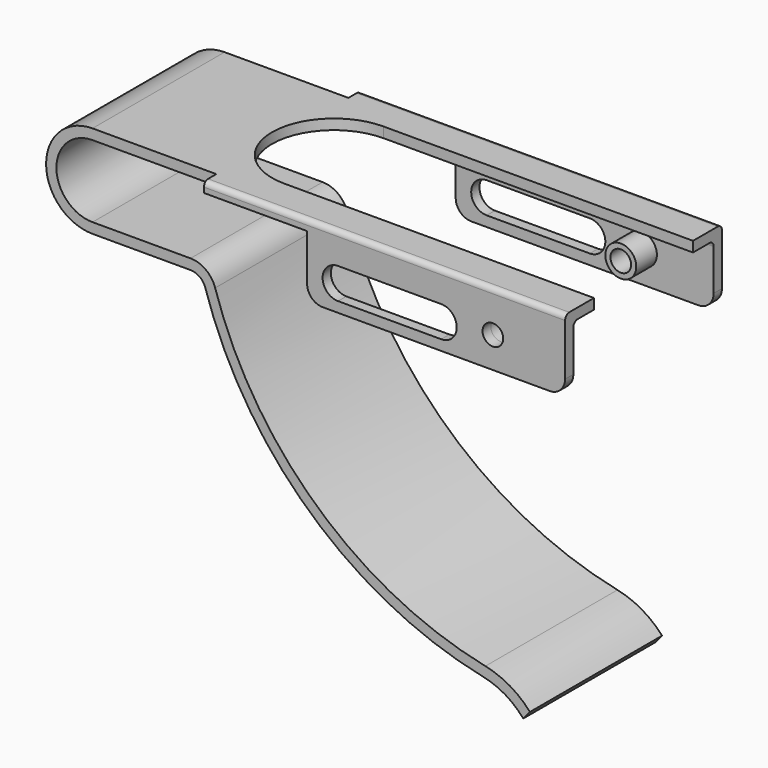
from build123d import *

# Parameters (mm, degrees)
F1_DEPTH  = 16
F2_W      = 70
F2_H      = 3
F3_DEPTH  = 2
F4_W      = 50
F4_H      = 14
F5_DEPTH  = 2
F6_R      = 1
F9_DEPTH  = 2
F11_DEPTH = 38.001
F13_D     = 4
F14_R     = 3
F14_R_2   = 2
F15_DEPTH = 5
F16_R     = 3


# Not quite as in the source:
# - a pattern or mirror of a feature is missing from the dataset's text; its kind, count and spacing are read off the source's solid


with BuildPart() as f1:
    # F0 (on Front) → F1 (new body)
    with BuildSketch(Plane.XZ):
        with BuildLine():
            Line((94, 9), (0, 9))
            ThreePointArc((0, 9), (-9, 0), (0, -9))
            Line((0, -9), (19, -9))
            ThreePointArc((19, -9), (20.7747485708, -9.5812673752), (21.8617615127, -11.0998216597))
            ThreePointArc((21.8617615127, -11.0998216597), (42.1784205856, -42.831899352), (75.7404983282, -59.9572702431))
            ThreePointArc((75.7404983282, -59.9572702431), (79.997153255, -61.6128288571), (83.4944279816, -64.5503541724))
            Line((83.4944279816, -64.5503541724), (84.7953295958, -63))
            ThreePointArc((84.7953295958, -63), (80.8735692863, -59.8084227638), (76.1517077584, -58))
            ThreePointArc((76.1517077584, -58), (43.5219099532, -41.3503338559), (23.7696025212, -10.4997027661))
            ThreePointArc((23.7696025212, -10.4997027661), (21.9579142847, -7.9687789586), (19, -7))
            Line((19, -7), (0, -7))
            ThreePointArc((0, -7), (-7, 0), (0, 7))
            Line((0, 7), (94, 7))
            Line((94, 7), (94, 9))
        make_face()
    extrude(amount=F1_DEPTH)

    # F2 (on face) → F3 (join)
    with BuildSketch(Plane.XY.offset(9)):
        with Locations((59, -17.5)):
            Rectangle(F2_W, F2_H)
    extrude(amount=-F3_DEPTH)

    # F4 (on face) → F5 (join)
    with BuildSketch(Plane.XZ.offset(19)):
        with Locations((69, 2)):
            Rectangle(F4_W, F4_H)
    extrude(amount=-F5_DEPTH)

    # F6
    f6_edges = [f1.edges().sort_by_distance(p)[0] for p in [
        (59, -19, 9),
        (69, -17, 7),
    ]]
    fillet(f6_edges, radius=F6_R)

    # F7: F1 across plane


with BuildPart() as f1_1:
    add(f1.part)
    add(f1.part.mirror(Plane.XZ))

    # F8 (on face) → F9 (cut)
    with BuildSketch(Plane.XY.offset(9)):
        with BuildLine():
            Line((94, 12), (34, 12))
            ThreePointArc((34, 12), (22, 0), (34, -12))
            Line((34, -12), (94, -12))
            Line((94, -12), (94, 12))
        make_face()
    extrude(amount=-F9_DEPTH, mode=Mode.SUBTRACT)

    # F10 (on face) → F11 (cut, through all)
    with BuildSketch(Plane.XZ.offset(19)):
        with BuildLine():
            ThreePointArc((50, 3), (47, 0), (50, -3))
            Line((50, -3), (70, -3))
            ThreePointArc((70, -3), (73, 0), (70, 3))
            Line((70, 3), (50, 3))
        make_face()
    extrude(amount=-F11_DEPTH, mode=Mode.SUBTRACT)

    # F13 (through all)
    with Locations(Plane.XZ.offset(19)):
        with Locations((80, 1)):
            Hole(F13_D / 2)

    # F14 (on face) → F15 (join)
    with BuildSketch(Plane(origin=(0, -17, 0), x_dir=(-1, 0, 0), z_dir=(0, 1, 0))):
        with Locations((-80, 1)):
            Circle(F14_R)
        with Locations((-80, 1)):
            Circle(F14_R_2, mode=Mode.SUBTRACT)
    f15 = extrude(amount=F15_DEPTH)

    # F15_copies: F15 across plane
    add(f15.mirror(Plane.ZX))

    # F16
    f16_edges = [f1_1.edges().sort_by_distance(p)[0] for p in [
        (94, -18, -5),
        (94, 18, -5),
        (44, 18, -5),
        (44, -18, -5),
    ]]
    fillet(f16_edges, radius=F16_R)


solid = f1_1.part
